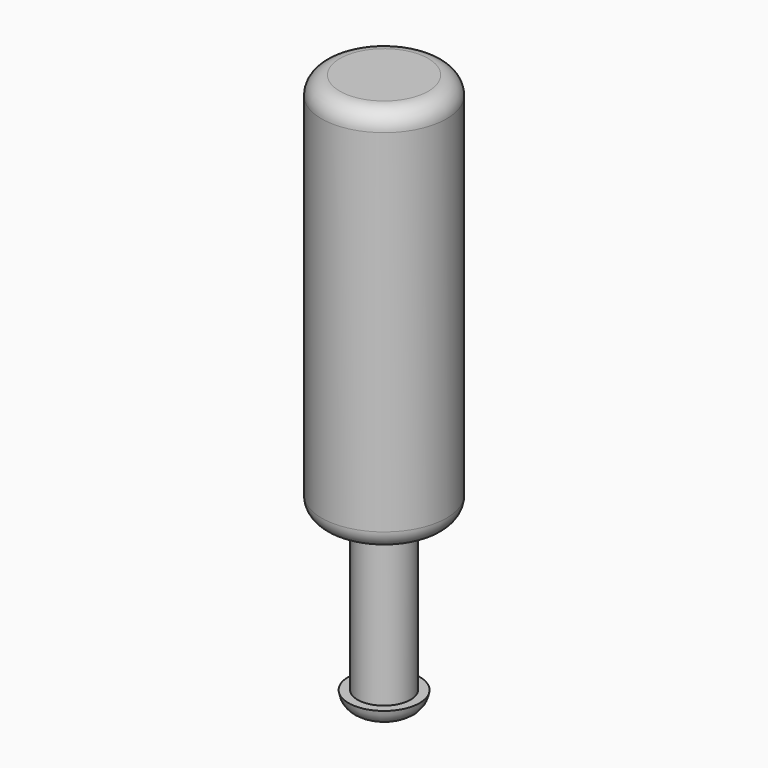
from build123d import *

# Parameters (mm, degrees)
F0_R     = 17.3493533367
F1_DEPTH = 107.62834
F2_R     = 5.08
F3_R     = 5.08
F4_R     = 7.3657213081
F5_DEPTH = 42.52659
F6_R     = 9.8562945963
F7_DEPTH = 4.6773


# Not quite as in the source:
# - a fillet or chamfer that OpenCascade refuses, or shapes differently, is made with other operations: its cross-section is extruded or revolved along the edge and cut away or added


with BuildPart() as f1:
    # F0 (on Top) → F1 (new body)
    with BuildSketch(Plane.XY):
        Circle(F0_R)
    extrude(amount=F1_DEPTH)

    # F2
    f2_edges = [f1.edges().sort_by_distance(p)[0] for p in [
        (-17.349353, 0, 107.62834),
    ]]
    fillet(f2_edges, radius=F2_R)

    # F3
    f3_edges = [f1.edges().sort_by_distance(p)[0] for p in [
        (-17.349353, 0, 0),
    ]]
    fillet(f3_edges, radius=F3_R)

    # F4 (on Top) → F5 (join)
    with BuildSketch(Plane.XY):
        Circle(F4_R)
    extrude(amount=-F5_DEPTH)

    # F6 (on face) → F7 (join)
    with BuildSketch(Plane(origin=(0, 0, -42.52659), x_dir=(1, 0, 0), z_dir=(0, 0, -1))):
        Circle(F6_R)
    extrude(amount=F7_DEPTH)

    # F8: fillet of radius 5.08 on 1 edges, made by hand

    # F8_s1 → F8_t2 (revolve, cut)
    with BuildSketch(Plane.XZ):
        with BuildLine():
            ThreePointArc((9.8562945963, -42.52659), (8.2390682978, -45.8556533901), (4.7922810981, -47.20389))
            Line((4.7922810981, -47.20389), (9.8562945963, -47.20389))
            Line((9.8562945963, -47.20389), (9.8562945963, -42.52659))
        make_face()
    revolve(axis=Axis((0, 0, -47.20389), (0, 0, -1)), mode=Mode.SUBTRACT)


solid = f1.part
